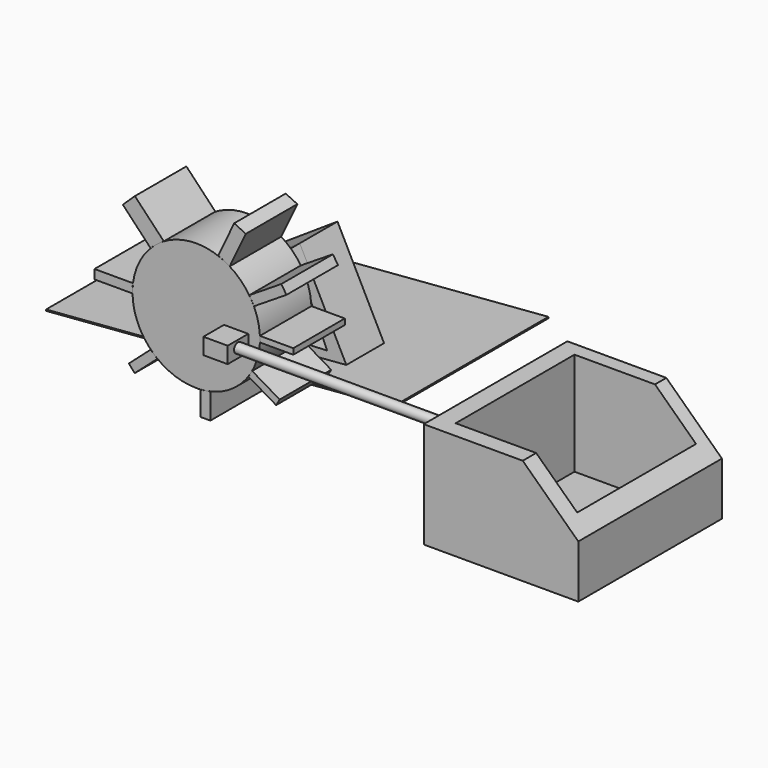
from build123d import *

# Parameters (mm, degrees)
F0_W      = 79.9928382039
F0_H      = 18.303444609
F1_DEPTH  = 50
F2_W      = 79.9928382039
F2_H      = 50
F3_DEPTH  = 18.304444609
F5_DEPTH  = 25
F6_W      = 135.3265494108
F6_H      = 100.133895874
F6_W_2    = 65.060867267
F6_H_2    = 18.303444609
F7_DEPTH  = 0.5
F9_DEPTH  = 25
F11_DEPTH = 25
F13_DEPTH = 25
F14_W     = 9.435325861
F14_H     = 6.3013508916
F15_DEPTH = 10
F16_R     = 1.8985138223
F17_DEPTH = 100
F18_W     = 69.6939403564
F18_H     = 41.1395505071
F18_R     = 1.8985138223
F19_DEPTH = 60
F20_W     = 47.1818447113
F20_H     = 57.6667264104
F21_DEPTH = 40
F23_DEPTH = 149.0666404197


# Not quite as in the source:
# - a feature names something its author has since deleted; it is built from what else it names


with BuildPart() as f1:
    # F0 (on Top) → F1 (new body)
    with BuildSketch(Plane.XY):
        Rectangle(F0_W, F0_H)
    extrude(amount=F1_DEPTH)

    # F2 (on face) → F3 (cut, through all)
    with BuildSketch(Plane.XZ.offset(9.1517223045)):
        with Locations((0, 25)):
            Rectangle(F2_W, F2_H)
        Polygon((35.7030183077, 11.4114070311), (-29.1499290615, 6.2141320668), (-36.3809205592, 11.4114070311), (17.6255404949, 47.1144206822), align=None, mode=Mode.SUBTRACT)
        Polygon((17.6255404949, 38.7535877526), (-29.1499290615, 11.4114070311), (28.2460581511, 13.8970594853), align=None)
    extrude(amount=-F3_DEPTH, mode=Mode.SUBTRACT)

    # F4 (on face) → F5 (join)
    with BuildSketch(Plane.XZ.offset(9.1517223045)):
        Polygon((14.1004873602, 44.7840509869), (17.6255404949, 38.7535877526), (20.7972230716, 40.8503484757), (17.6255404949, 47.1144206822), align=None)
    extrude(amount=F5_DEPTH)

    # F8 (on face) → F9 (join)
    with BuildSketch(Plane.XZ.offset(34.1517223045)):
        Polygon((20.7972230716, 40.8503484757), (19.8864468458, 42.6491312683), (15.3484355118, 42.6491312683), (17.6255404949, 38.7535877526), align=None)
        Polygon((15.3484355118, 42.6491312683), (19.8864468458, 42.6491312683), (17.6255404949, 47.1144206822), (14.1004873602, 44.7840509869), align=None)
        with BuildLine():
            Line((19.8864468458, 42.6491312683), (42.1685310007, 42.6491312683))
            ThreePointArc((42.1685310007, 42.6491312683), (17.4249261618, 67.3927361072), (-7.3186786772, 42.6491312683))
            Line((-7.3186786772, 42.6491312683), (15.3484355118, 42.6491312683))
            Line((15.3484355118, 42.6491312683), (14.1004873602, 44.7840509869))
            Line((14.1004873602, 44.7840509869), (17.6255404949, 47.1144206822))
            Line((17.6255404949, 47.1144206822), (19.8864468458, 42.6491312683))
        make_face()
        with BuildLine():
            ThreePointArc((-7.3186786772, 42.6491312683), (17.4249261618, 17.9055264293), (42.1685310007, 42.6491312683))
            Line((42.1685310007, 42.6491312683), (19.8864468458, 42.6491312683))
            Line((19.8864468458, 42.6491312683), (20.7972230716, 40.8503484757))
            Line((20.7972230716, 40.8503484757), (17.6255404949, 38.7535877526))
            Line((17.6255404949, 38.7535877526), (15.3484355118, 42.6491312683))
            Line((15.3484355118, 42.6491312683), (-7.3186786772, 42.6491312683))
        make_face()
    extrude(amount=F9_DEPTH)

    # F14 (on face) → F15 (join)
    with BuildSketch(Plane.XZ.offset(59.1517223045)):
        with Locations((32.9205654562, 39.8556888103)):
            Rectangle(F14_W, F14_H)
    extrude(amount=F15_DEPTH)

    # F16 (on face) → F17 (join)
    with BuildSketch(Plane.YZ.offset(37.6382283866)):
        with Locations((-64.1517223045, 40.2767546475)):
            Circle(F16_R)
    extrude(amount=F17_DEPTH)


with BuildPart() as f7:
    # F6 (on face) → F7 (new body)
    with BuildSketch(Plane(origin=(-0.6808343292, 0, 8.4956276551), x_dir=(0.9968042249, 0, 0.0798832721), z_dir=(0.0798832721, 0, -0.9968042249))):
        Rectangle(F6_W, F6_H)
        with Locations((3.9700663915, 0)):
            Rectangle(F6_W_2, F6_H_2, mode=Mode.SUBTRACT)
    extrude(amount=F7_DEPTH)

    # F11 (cut): a face of the model
    f11_faces = [f7.faces().sort_by_distance(p)[0] for p in [
        (-0.6608635112, -50.066947937, 8.2464265988),
    ]]
    extrude(f11_faces, amount=-F11_DEPTH, mode=Mode.SUBTRACT)


with BuildPart() as f13:
    # F12 (on face) → F13 (new body)
    with BuildSketch(Plane.XZ.offset(59.1517223045)):
        with BuildLine():
            ThreePointArc((25.9287375384, 65.8855503662), (28.2297677146, 64.9089915428), (30.4205267746, 63.7052549651))
            Line((30.4205267746, 63.7052549651), (36.6799546023, 76.8704908801))
            Line((36.6799546023, 76.8704908801), (32.170843333, 79.0143534541))
            Line((32.170843333, 79.0143534541), (25.9287375384, 65.8855503662))
        make_face()
    extrude(amount=-F13_DEPTH)


with BuildPart() as f13b:
    # F12 (on face) → F13, piece 2 (new body)
    with BuildSketch(Plane.XZ.offset(59.1517223045)):
        with BuildLine():
            ThreePointArc((38.0318597301, 56.345856035), (38.9903960982, 54.7807629329), (39.8302887258, 53.1489269235))
            Line((39.8302887258, 53.1489269235), (52.4495742528, 61.130350821))
            Line((52.4495742528, 61.130350821), (50.491463393, 64.2262846231))
            Line((50.491463393, 64.2262846231), (38.0318597301, 56.345856035))
        make_face()
    extrude(amount=-F13_DEPTH)


with BuildPart() as f13c:
    # F12 (on face) → F13, piece 3 (new body)
    with BuildSketch(Plane.XZ.offset(59.1517223045)):
        with BuildLine():
            Line((49.8318262398, 24.5164651424), (39.1453309961, 30.7971274605))
            ThreePointArc((39.1453309961, 30.7971274605), (38.4514582478, 29.6057065315), (37.6923008836, 28.4547837204))
            Line((37.6923008836, 28.4547837203), (48.4355733395, 22.1407523238))
            Line((48.4355733395, 22.1407523238), (49.8318262398, 24.5164651424))
        make_face()
    extrude(amount=-F13_DEPTH)


with BuildPart() as f13d:
    # F12 (on face) → F13, piece 4 (new body)
    with BuildSketch(Plane.XZ.offset(59.1517223045)):
        with BuildLine():
            ThreePointArc((-7.3145034198, 42.1945936978), (-7.2829121383, 43.9790586964), (-7.122774146, 45.7566045225))
            Line((-7.122774146, 45.7566045225), (-22.0680162311, 45.7566045225))
            Line((-22.0680162311, 45.7566045225), (-22.0680162311, 42.1945936978))
            Line((-22.0680162311, 42.1945936978), (-7.3145034198, 42.1945936978))
        make_face()
    extrude(amount=-F13_DEPTH)


with BuildPart() as f13e:
    # F12 (on face) → F13, piece 5 (new body)
    with BuildSketch(Plane.XZ.offset(59.1517223045)):
        with BuildLine():
            Line((55.1088824868, 43.7777079642), (42.1427799332, 43.7777079642))
            ThreePointArc((42.1427799332, 43.7777079642), (42.1620923961, 43.2135664895), (42.1685310007, 42.6491312683))
            ThreePointArc((42.1685310007, 42.6491312683), (42.1622558216, 42.0919044519), (42.1434334673, 41.5349602699))
            Line((42.1434334673, 41.5349602699), (55.1088824868, 41.5349602699))
            Line((55.1088824868, 41.5349602699), (55.1088824868, 43.7777079642))
        make_face()
    extrude(amount=-F13_DEPTH)


with BuildPart() as f13f:
    # F12 (on face) → F13, piece 6 (new body)
    with BuildSketch(Plane.XZ.offset(59.1517223045)):
        with BuildLine():
            Line((22.9188613594, 8.5533810779), (22.9188613594, 18.5231565425))
            ThreePointArc((22.9188613594, 18.5231565425), (21.0169117184, 18.1676358036), (19.0929975361, 17.961816341))
            Line((19.0929975361, 17.961816341), (19.0929975361, 8.5533810779))
            Line((19.0929975361, 8.5533810779), (22.9188613594, 8.5533810779))
        make_face()
    extrude(amount=-F13_DEPTH)


with BuildPart() as f13g:
    # F12 (on face) → F13, piece 7 (new body)
    with BuildSketch(Plane.XZ.offset(59.1517223045)):
        with BuildLine():
            Line((-6.4659747203, 15.2110734288), (2.3657253742, 23.0158316968))
            ThreePointArc((2.3657253742, 23.0158316968), (1.0278812114, 24.1185377181), (-0.2294625715, 25.3122186573))
            Line((-0.2294625715, 25.3122186573), (-8.7434565648, 17.7882239223))
            Line((-8.7434565648, 17.7882239223), (-6.4659747203, 15.2110734288))
        make_face()
    extrude(amount=-F13_DEPTH)


with BuildPart() as f13h:
    # F12 (on face) → F13, piece 8 (new body)
    with BuildSketch(Plane.XZ.offset(59.1517223045)):
        with BuildLine():
            ThreePointArc((-0.2773562415, 59.9371380401), (2.1540120961, 62.1182135277), (4.8514824982, 63.9600321142))
            Line((4.8514824982, 63.9600321142), (-6.3894838095, 75.7631883025))
            Line((-6.3894838095, 75.7631883025), (-11.0599229864, 71.3152043402))
            Line((-11.0599229864, 71.3152043402), (-0.2773562415, 59.9371380401))
        make_face()
    extrude(amount=-F13_DEPTH)


with BuildPart() as f19:
    # F18 (on face) → F19 (new body)
    with BuildSketch(Plane.YZ.offset(137.6382283866)):
        with Locations((-64.1517223045, 40.2767546475)):
            Rectangle(F18_W, F18_H)
        with Locations((-64.1517223045, 40.2767546475)):
            Circle(F18_R, mode=Mode.SUBTRACT)
        with Locations((-64.1517223045, 40.2767546475)):
            Circle(F18_R)
    extrude(amount=F19_DEPTH)

    # F20 (on face) → F21 (cut)
    with BuildSketch(Plane.XY.offset(60.846529901)):
        with Locations((168.3957129717, -63.6372715235)):
            Rectangle(F20_W, F20_H)
    extrude(amount=-F21_DEPTH, mode=Mode.SUBTRACT)

    # F22 (on face) → F23 (cut, through all)
    with BuildSketch(Plane.XZ.offset(98.9986924827)):
        Polygon((197.6382283866, 60.846529901), (176.0575026274, 60.846529901), (197.6382283866, 40.2767546475), align=None)
    extrude(amount=-F23_DEPTH, mode=Mode.SUBTRACT)


solid = Compound([f1.part, f7.part, f13.part, f13b.part, f13c.part, f13d.part, f13e.part, f13f.part, f13g.part, f13h.part, f19.part])
